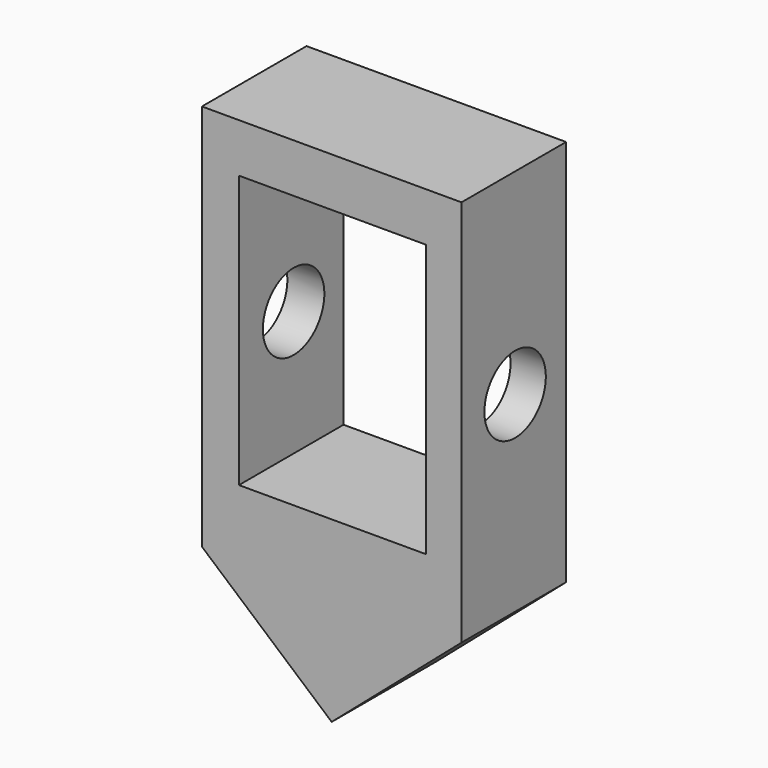
from build123d import *

# Parameters (mm, degrees)
F1_DEPTH = 40.64
F2_W     = 58.1915168336
F2_H     = 84.6826420166
F3_DEPTH = 100.584
F4_DEPTH = 25.4
F5_R     = 11.938
F6_DEPTH = 25.4
F7_R     = 11.938
F8_DEPTH = 25.4


# Not quite as in the source:
# - a feature names something its author has since deleted; it is built from what else it names


with BuildPart() as f1:
    # F0 (on Front) → F1 (new body)
    with BuildSketch(Plane.XZ):
        Polygon((5.0445693985, -63.1324924332), (45.3936140645, -28.3097998209), (45.3936140645, 92.1692103148), (-35.2877192199, 92.1692103148), (-35.2877192199, -28.3036921173), align=None)
    extrude(amount=F1_DEPTH)

    # F2 (on face) → F3 (cut)
    with BuildSketch(Plane.XZ.offset(40.64)):
        with Locations((5.3103963967, 34.6377051901)):
            Rectangle(F2_W, F2_H)
    extrude(amount=-F3_DEPTH, mode=Mode.SUBTRACT)

    # F2 (on face) → F4 (cut)
    with BuildSketch(Plane.XZ.offset(40.64)):
        with Locations((5.3103963967, 34.6377051901)):
            Rectangle(F2_W, F2_H)
    extrude(amount=-F4_DEPTH, mode=Mode.SUBTRACT)

    # F5 (on face) → F6 (cut)
    with BuildSketch(Plane(origin=(-35.2877192199, 0, 0), x_dir=(0, -1, 0), z_dir=(-1, 0, 0))):
        with Locations((19.3923822703, 31.1755515458)):
            Circle(F5_R)
    extrude(amount=-F6_DEPTH, mode=Mode.SUBTRACT)

    # F7 (on face) → F8 (cut)
    with BuildSketch(Plane.YZ.offset(45.3936140645)):
        with Locations((-19.7985949944, 31.1684036463)):
            Circle(F7_R)
    extrude(amount=-F8_DEPTH, mode=Mode.SUBTRACT)


solid = f1.part
